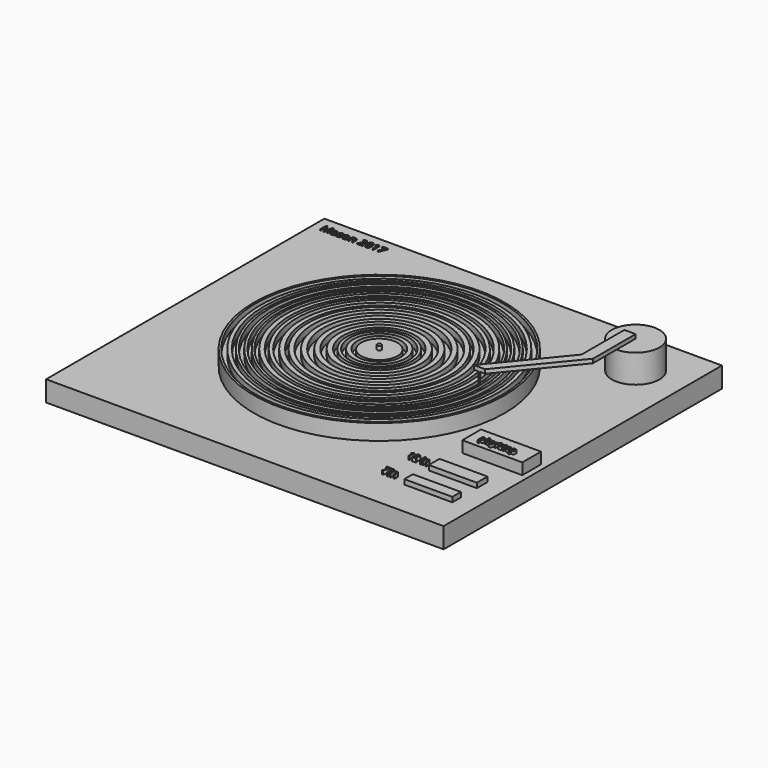
from build123d import *

# Parameters (mm, degrees)
F0_W            = 98.6984670162
F0_H            = 86.3612965102
F1_DEPTH        = 5.08
F2_R            = 31.156005255
F3_DEPTH        = 2.3
F4_R            = 31.156005255
F4_R_2          = 30.6611592983
F4_R_3          = 29.4866578201
F4_R_4          = 28.6056057905
F4_R_5          = 27.8142144613
F4_R_6          = 27.2510988872
F4_R_7          = 26.1923924199
F4_R_8          = 25.5781961877
F4_R_9          = 24.7586671221
F4_R_10         = 24.2262392051
F4_R_11         = 23.29553032
F4_R_12         = 22.2252370843
F4_R_13         = 21.4545488022
F4_R_14         = 20.5897211573
F4_R_15         = 19.4222273733
F4_R_16         = 18.2918713325
F4_R_17         = 17.6011317981
F4_R_18         = 16.4888289816
F4_R_19         = 15.1890669019
F4_R_20         = 13.9911540863
F4_R_21         = 12.6250610934
F4_R_22         = 11.4428912901
F4_R_23         = 10.2118226797
F4_R_24         = 8.9722442964
F4_R_25         = 8.1242020252
F4_R_26         = 7.4171270481
F4_R_27         = 6.4477778527
F4_R_28         = 5.420549124
F5_DEPTH        = 1.6
F6_R            = 5.9132088967
F7_DEPTH        = 7
F9_DEPTH        = 1
F11_DEPTH       = 0.4
F12_R           = 4.5011682677
F13_DEPTH       = 1.5
F14_R           = 0.5209758674
F15_DEPTH       = 1
F16_W           = 11.9140781462
F16_H           = 3.3094678074
F16_H_2         = 2.6475712657
F17_DEPTH       = 1.2
F18_TEXT_SIZE   = 2.5280596068
F18_TEXT_SIZE_2 = 2.2982376524
F19_DEPTH       = 0.9
F20_W           = 14.8925930262
F20_H           = 5.7915654033
F21_DEPTH       = 2.8
F22_TEXT_SIZE   = 2.0432040199
F23_DEPTH       = 0.7
F24_TEXT_SIZE   = 2.7578841481
F25_DEPTH       = 0.2


# Not quite as in the source:
# - Text() gives the source's letters only with a copy of the font that has no kerning and outlines rounded to 1/6400 em; it was checked with that copy


with BuildPart() as f1:
    # F0 (on Top) → F1 (new body)
    with BuildSketch(Plane.XY):
        with Locations((2.190053463, -1.2775995013)):
            Rectangle(F0_W, F0_H)
    extrude(amount=F1_DEPTH)

    # F2 (on face) → F3 (join)
    with BuildSketch(Plane.XY.offset(5.08)):
        Circle(F2_R)
    extrude(amount=F3_DEPTH)

    # F4 (on face) → F5 (join)
    with BuildSketch(Plane.XY.offset(7.38)):
        Circle(F4_R)
        Circle(F4_R_2, mode=Mode.SUBTRACT)
        Circle(F4_R_3)
        Circle(F4_R_4, mode=Mode.SUBTRACT)
        Circle(F4_R_5)
        Circle(F4_R_6, mode=Mode.SUBTRACT)
        Circle(F4_R_7)
        Circle(F4_R_8, mode=Mode.SUBTRACT)
        Circle(F4_R_9)
        Circle(F4_R_10, mode=Mode.SUBTRACT)
        Circle(F4_R_11)
        Circle(F4_R_12, mode=Mode.SUBTRACT)
        Circle(F4_R_13)
        Circle(F4_R_14, mode=Mode.SUBTRACT)
        Circle(F4_R_15)
        Circle(F4_R_16, mode=Mode.SUBTRACT)
        Circle(F4_R_17)
        Circle(F4_R_18, mode=Mode.SUBTRACT)
        Circle(F4_R_19)
        Circle(F4_R_20, mode=Mode.SUBTRACT)
        Circle(F4_R_21)
        Circle(F4_R_22, mode=Mode.SUBTRACT)
        Circle(F4_R_23)
        Circle(F4_R_24, mode=Mode.SUBTRACT)
        Circle(F4_R_25)
        Circle(F4_R_26, mode=Mode.SUBTRACT)
        Circle(F4_R_27)
        Circle(F4_R_28, mode=Mode.SUBTRACT)
    extrude(amount=F5_DEPTH)

    # F6 (on face) → F7 (join)
    with BuildSketch(Plane.XY.offset(5.08)):
        with Locations((39.8352257907, 29.7486409545)):
            Circle(F6_R)
    extrude(amount=F7_DEPTH)

    # F8 (on face) → F9 (join)
    with BuildSketch(Plane.XY.offset(12.08)):
        with BuildLine():
            Line((39.8352257907, 16.5107790381), (39.8352257907, 23.8354320578))
            ThreePointArc((39.8352257907, 23.8354320578), (38.3920917226, 24.0142357092), (37.0362326503, 24.5398333313))
            Line((37.0362326503, 24.5398333313), (37.0362326503, 16.5107790381))
            Line((37.0362326503, 16.5107790381), (23.4674233943, 0))
            Line((23.4674233943, 0), (26.2664165348, 0))
            Line((26.2664165348, 0), (39.8352257907, 16.5107790381))
        make_face()
        with BuildLine():
            Line((39.8352257907, 23.8354320578), (39.8352257907, 29.7486409545))
            Line((39.8352257907, 29.7486409545), (37.0362326503, 29.7486409545))
            Line((37.0362326503, 29.7486409545), (37.0362326503, 24.5398333313))
            ThreePointArc((37.0362326503, 24.5398333313), (38.3920917226, 24.0142357092), (39.8352257907, 23.8354320578))
        make_face()
    extrude(amount=F9_DEPTH)

    # F12 (on face) → F13 (join)
    with BuildSketch(Plane.XY.offset(7.38)):
        Circle(F12_R)
    extrude(amount=F13_DEPTH)

    # F14 (on face) → F15 (join)
    with BuildSketch(Plane.XY.offset(8.88)):
        Circle(F14_R)
    extrude(amount=F15_DEPTH)

    # F16 (on face) → F17 (join)
    with BuildSketch(Plane.XY.offset(5.08)):
        with Locations((40.6625922769, -26.3468036428)):
            Rectangle(F16_W, F16_H)
        with Locations((40.6625922769, -34.2895202339)):
            Rectangle(F16_W, F16_H_2)
    extrude(amount=F17_DEPTH)

    # F18 (on face) → F19 (join)
    with BuildSketch(Plane.XY.offset(5.08)):
        with Locations((28.2520949841, -34.9514111876)):
            Text('7in', F18_TEXT_SIZE, font='Open Sans', text_align=(TextAlign.LEFT, TextAlign.BOTTOM))
        with Locations((28.2520949841, -27.0086936653)):
            Text('12 in', F18_TEXT_SIZE_2, font='Open Sans', text_align=(TextAlign.LEFT, TextAlign.BOTTOM))
    extrude(amount=F19_DEPTH)

    # F20 (on face) → F21 (join)
    with BuildSketch(Plane.XY.offset(5.08)):
        with Locations((42.6482707262, -15.3428288177)):
            Rectangle(F20_W, F20_H)
    extrude(amount=F21_DEPTH)

    # F22 (on face) → F23 (join)
    with BuildSketch(Plane.XY.offset(7.88)):
        with Locations((38.0816571414, -16.813935712)):
            Text('play/stop', F22_TEXT_SIZE, font='Open Sans', text_align=(TextAlign.LEFT, TextAlign.BOTTOM))
    extrude(amount=F23_DEPTH)

    # F24 (on face) → F25 (join)
    with BuildSketch(Plane.XY.offset(5.08)):
        with Locations((-45.0525693595, 37.5258885324)):
            Text('Mason 2017', F24_TEXT_SIZE, font='Open Sans', text_align=(TextAlign.LEFT, TextAlign.BOTTOM))
    extrude(amount=F25_DEPTH)


with BuildPart() as f11:
    # F10 (on face) → F11 (new body)
    with BuildSketch(Plane.XZ):
        Polygon((24.653095752, 8.9536914602), (24.8669199646, 12.08), (24.653095752, 12.08), align=None)
    extrude(amount=-F11_DEPTH)


solid = Compound([f1.part, f11.part])
